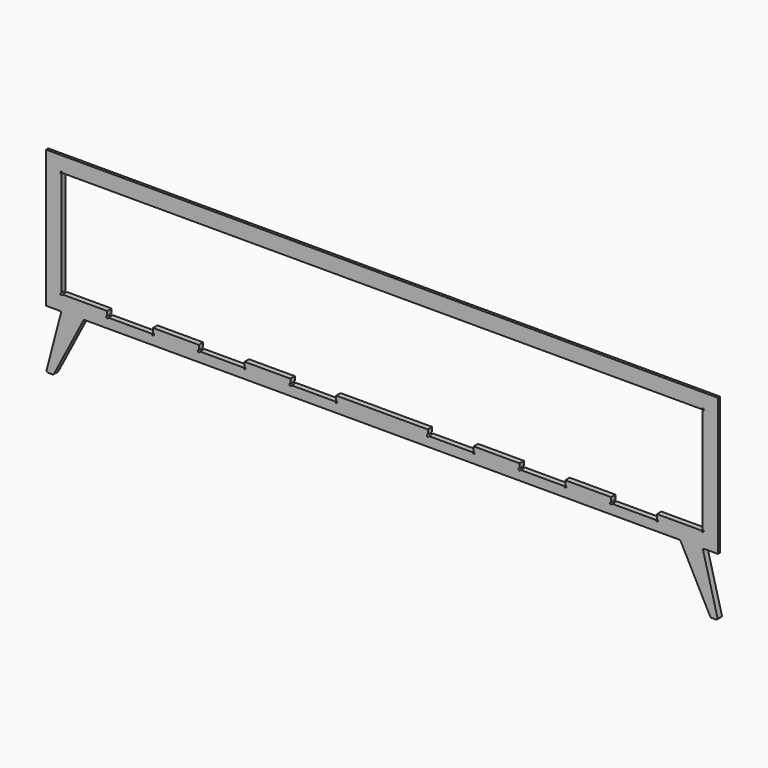
from build123d import *

# Parameters (mm, degrees)
F0_W     = 9
F0_H     = 9
F0_H_2   = 441
F1_DEPTH = 18
F2_DEPTH = 9


# Not quite as in the source:
# - ends of sketch curves that miss each other by under 0.0002 mm in the source are joined


with BuildPart() as f1:
    # F0 (on Front) → F1 (new body)
    with BuildSketch(Plane.XZ):
        with Locations((-1095.5, 71.3756743552)):
            Rectangle(F0_W, F0_H)
        with BuildLine():
            Line((0, 66.8756743552), (-1091, 66.8756743552))
            Line((-1091, 66.8756743552), (-1091, -374.1243256448))
            Line((-1091, -374.1243256448), (-1055, -374.1243256448))
            ThreePointArc((-1055, -374.1243256448), (-1054.8038113281, -374.1191399972), (-1054.6076226562, -374.1243256448))
            Line((-1054.6076226562, -374.1243256448), (-973.3476458471, -374.1243256448))
            Line((-973.3476458471, -374.1243256448), (0, -374.1243256448))
            Line((0, -374.1243256448), (973.3476458471, -374.1243256448))
            Line((973.3476458471, -374.1243256448), (1054.6076226562, -374.1243256448))
            ThreePointArc((1054.6076226562, -374.1243256448), (1054.8038113281, -374.1191399972), (1055, -374.1243256448))
            Line((1055, -374.1243256448), (1091, -374.1243256448))
            Line((1091, -374.1243256448), (1091, -365.1243256448))
            Line((1091, -365.1243256448), (1091, -365.0378882885))
            Line((1091, -365.0378882885), (1091, 66.8756743552))
            Line((1091, 66.8756743552), (0, 66.8756743552))
        make_face()
        with BuildLine():
            Line((-1050, -320.6243256448), (-1050, 22.3756743552))
            ThreePointArc((-1050, 22.3756743552), (-1052.4748737342, 28.3505480894), (-1046.5, 25.8756743552))
            Line((-1046.5, 25.8756743552), (0, 25.8756743552))
            Line((0, 25.8756743552), (1046.5, 25.8756743552))
            ThreePointArc((1046.5, 25.8756743552), (1052.4748737342, 28.3505480894), (1050, 22.3756743552))
            Line((1050, 22.3756743552), (1050, -320.6243256448))
            ThreePointArc((1050, -320.6243256448), (1052.4748737342, -326.5991993789), (1046.5, -324.1243256448))
            Line((1046.5, -324.1243256448), (900, -324.1243256448))
            Line((900, -324.1243256448), (900, -338.6243256448))
            ThreePointArc((900, -338.6243256448), (902.4748737342, -344.5991993789), (896.5, -342.1243256448))
            Line((896.5, -342.1243256448), (753.5000238419, -342.1243256448))
            ThreePointArc((753.5000238419, -342.1243256448), (747.5251501077, -344.5991993789), (750.0000238419, -338.6243256448))
            Line((750.0000238419, -338.6243256448), (750.0000238419, -324.1243256448))
            Line((750.0000238419, -324.1243256448), (600.0000238419, -324.1243256448))
            Line((600.0000238419, -324.1243256448), (600, -338.6243256448))
            ThreePointArc((600, -338.6243256448), (602.4748737342, -344.5991993789), (596.5, -342.1243256448))
            Line((596.5, -342.1243256448), (453.5000238419, -342.1243256448))
            ThreePointArc((453.5000238419, -342.1243256448), (447.5251501077, -344.5991993789), (450.0000238419, -338.6243256448))
            Line((450.0000238419, -338.6243256448), (450.0000238419, -324.1243256448))
            Line((450.0000238419, -324.1243256448), (300.0000238419, -324.1243256448))
            Line((300.0000238419, -324.1243256448), (300, -338.6243256448))
            ThreePointArc((300, -338.6243256448), (302.4748737342, -344.5991993789), (296.5, -342.1243256448))
            Line((296.5, -342.1243256448), (153.5000238419, -342.1243256448))
            ThreePointArc((153.5000238419, -342.1243256448), (147.5251501077, -344.5991993789), (150.0000238419, -338.6243256448))
            Line((150.0000238419, -338.6243256448), (150.0000238419, -324.1243256448))
            Line((150.0000238419, -324.1243256448), (2.38419e-05, -324.1243256448))
            Line((2.38419e-05, -324.1243256448), (-150.0000238419, -324.1243256448))
            Line((-150.0000238419, -324.1243256448), (-150.0000238419, -338.6243256448))
            ThreePointArc((-150.0000238419, -338.6243256448), (-147.5251501077, -344.5991993789), (-153.5000238419, -342.1243256448))
            Line((-153.5000238419, -342.1243256448), (-296.5, -342.1243256448))
            ThreePointArc((-296.5, -342.1243256448), (-302.4748737342, -344.5991993789), (-300, -338.6243256448))
            Line((-300, -338.6243256448), (-300, -324.1243256448))
            Line((-300, -324.1243256448), (-450.0000238419, -324.1243256448))
            Line((-450.0000238419, -324.1243256448), (-450.0000238419, -338.6243256448))
            ThreePointArc((-450.0000238419, -338.6243256448), (-447.5251501077, -344.5991993789), (-453.5000238419, -342.1243256448))
            Line((-453.5000238419, -342.1243256448), (-596.5, -342.1243256448))
            ThreePointArc((-596.5, -342.1243256448), (-602.4748737342, -344.5991993789), (-600, -338.6243256448))
            Line((-600, -338.6243256448), (-600, -324.1243256448))
            Line((-600, -324.1243256448), (-750.0000238419, -324.1243256448))
            Line((-750.0000238419, -324.1243256448), (-750.0000238419, -338.6243256448))
            ThreePointArc((-750.0000238419, -338.6243256448), (-747.5251501077, -344.5991993789), (-753.5000238419, -342.1243256448))
            Line((-753.5000238419, -342.1243256448), (-896.5, -342.1243256448))
            ThreePointArc((-896.5, -342.1243256448), (-902.4748737342, -344.5991993789), (-900, -338.6243256448))
            Line((-900, -338.6243256448), (-900, -324.1243256448))
            Line((-900, -324.1243256448), (-1046.5, -324.1243256448))
            ThreePointArc((-1046.5, -324.1243256448), (-1052.4748737342, -326.5991993789), (-1050, -320.6243256448))
        make_face(mode=Mode.SUBTRACT)
        with BuildLine():
            Line((-973.3476458471, -374.1243256448), (-1054.6076226562, -374.1243256448))
            ThreePointArc((-1054.6076226562, -374.1243256448), (-1051.7483407187, -375.721921149), (-1051.265639742, -378.9614896944))
            Line((-1051.265639742, -378.9614896944), (-1098.3606008427, -558.954299013))
            ThreePointArc((-1098.3606008427, -558.954299013), (-1097.4812264988, -563.2754093644), (-1093.523436793, -565.219938755))
            Line((-1093.523436793, -565.219938755), (-1078.8076104242, -565.219938755))
            ThreePointArc((-1078.8076104242, -565.219938755), (-1076.2129629213, -564.4940239596), (-1074.371712623, -562.5270604893))
            Line((-1074.371712623, -562.5270604893), (-977.7835436484, -376.8172039105))
            ThreePointArc((-977.7835436484, -376.8172039105), (-975.94229335, -374.8502404402), (-973.3476458471, -374.1243256448))
        make_face()
        Polygon((1100, 66.8756743552), (1091, 66.8756743552), (1091, -365.0378882885), (1091, -365.1243256448), (1091, -374.1243256448), (1100, -374.1243256448), align=None)
        Polygon((0, 75.8756743552), (-1091, 75.8756743552), (-1091, 66.8756743552), (0, 66.8756743552), (1091, 66.8756743552), (1091, 75.8756743552), align=None)
        with Locations((-1095.5, -153.6243256448)):
            Rectangle(F0_W, F0_H_2)
        with Locations((1095.5, 71.3756743552)):
            Rectangle(F0_W, F0_H)
        with BuildLine():
            Line((1054.6076226562, -374.1243256448), (973.3476458471, -374.1243256448))
            ThreePointArc((973.3476458471, -374.1243256448), (975.94229335, -374.8502404402), (977.7835436484, -376.8172039105))
            Line((977.7835436484, -376.8172039105), (1074.371712623, -562.5270604893))
            ThreePointArc((1074.371712623, -562.5270604893), (1076.2129629213, -564.4940239596), (1078.8076104242, -565.219938755))
            Line((1078.8076104242, -565.219938755), (1093.523436793, -565.219938755))
            ThreePointArc((1093.523436793, -565.219938755), (1097.4812264988, -563.2754093644), (1098.3606008427, -558.954299013))
            Line((1098.3606008427, -558.954299013), (1051.265639742, -378.9614896944))
            ThreePointArc((1051.265639742, -378.9614896944), (1051.7483407187, -375.721921149), (1054.6076226562, -374.1243256448))
        make_face()
    extrude(amount=F1_DEPTH)

    # F0 (on Front) → F2 (cut)
    with BuildSketch(Plane.XZ):
        Polygon((0, 75.8756743552), (-1091, 75.8756743552), (-1091, 66.8756743552), (0, 66.8756743552), (1091, 66.8756743552), (1091, 75.8756743552), align=None)
        with Locations((1095.5, 71.3756743552)):
            Rectangle(F0_W, F0_H)
        with Locations((-1095.5, -153.6243256448)):
            Rectangle(F0_W, F0_H_2)
        with Locations((-1095.5, 71.3756743552)):
            Rectangle(F0_W, F0_H)
        Polygon((1100, 66.8756743552), (1091, 66.8756743552), (1091, -365.0378882885), (1091, -365.1243256448), (1091, -374.1243256448), (1100, -374.1243256448), align=None)
    extrude(amount=F2_DEPTH, mode=Mode.SUBTRACT)


solid = f1.part
